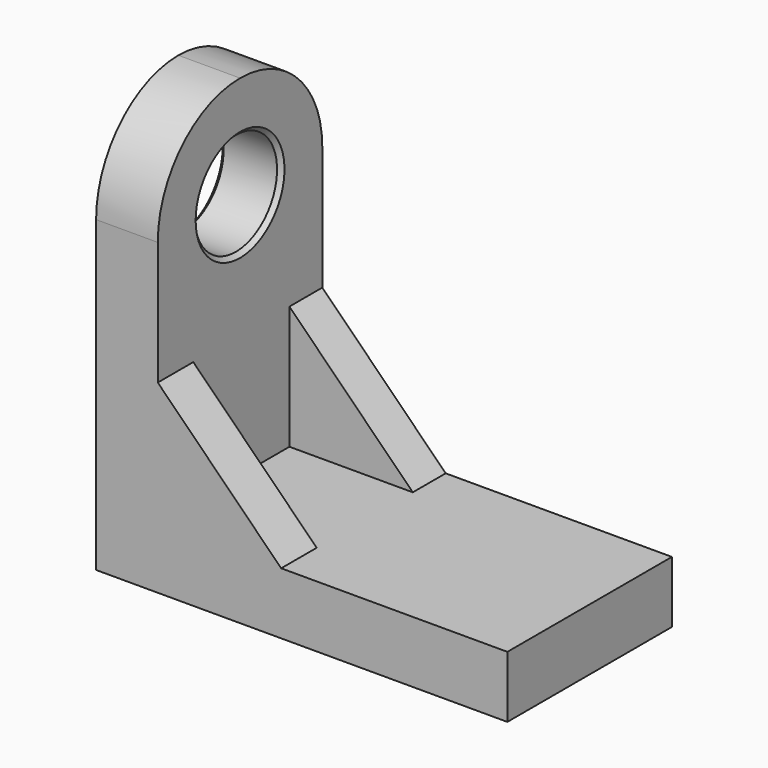
from build123d import *

# Parameters (mm, degrees)
F0_W     = 100
F0_H     = 50
F1_DEPTH = 15
F2_W     = 15
F2_H     = 50
F3_DEPTH = 85
F4_W     = 30
F4_H     = 10.7893505692
F4_H_2   = 10
F5_DEPTH = 30
F6_SIZE  = 29.99999
F7_R     = 12.5
F8_R     = 12.5
F9_DEPTH = 25
F10_R    = 24.99999
F11_SIZE = 1


# Not quite as in the source:
# - a fillet or chamfer is up to 0.001 mm smaller than in the source, because OpenCascade refuses the exact size


with BuildPart() as f1:
    # F0 (on Top) → F1 (new body)
    with BuildSketch(Plane.XY):
        with Locations((1.2109465897, -8.8487002536)):
            Rectangle(F0_W, F0_H)
    extrude(amount=F1_DEPTH)

    # F2 (on face) → F3 (join)
    with BuildSketch(Plane.XY.offset(15)):
        with Locations((-41.2890534103, -8.8487002536)):
            Rectangle(F2_W, F2_H)
    extrude(amount=F3_DEPTH)

    # F4 (on face) → F5 (join)
    with BuildSketch(Plane.XY.offset(15)):
        with Locations((-18.7890534103, -28.454024969)):
            Rectangle(F4_W, F4_H)
        with Locations((-18.7890534103, 11.1512997464)):
            Rectangle(F4_W, F4_H_2)
    extrude(amount=F5_DEPTH)

    # F6 (size 30 in the source; OpenCascade refuses exactly that, so slightly less here)
    f6_edges = [f1.edges().sort_by_distance(p)[0] for p in [
        (-3.789053, 11.1513, 45),
        (-3.789053, -28.454025, 45),
    ]]
    chamfer(f6_edges, length=F6_SIZE)

    # F7 (on face) + F8 (on face) → F9 (cut)
    with BuildSketch(Plane(origin=(-48.7890534103, 0, 0), x_dir=(0, -1, 0), z_dir=(-1, 0, 0))):
        with Locations((8.8487002536, 75)):
            Circle(F7_R)
    with BuildSketch(Plane(origin=(-48.7890534103, 0, 0), x_dir=(0, -1, 0), z_dir=(-1, 0, 0))):
        with Locations((8.8487002536, 75)):
            Circle(F8_R)
    extrude(amount=-F9_DEPTH, mode=Mode.SUBTRACT)

    # F10 (radius 25 in the source; OpenCascade refuses exactly that, so slightly less here)
    f10_edges = [f1.edges().sort_by_distance(p)[0] for p in [
        (-41.289053, 16.1513, 100),
        (-41.289053, -33.8487, 100),
    ]]
    fillet(f10_edges, radius=F10_R)

    # F11
    f11_edges = [f1.edges().sort_by_distance(p)[0] for p in [
        (-33.789053, 3.6513, 75),
        (-48.789053, 3.6513, 75),
    ]]
    chamfer(f11_edges, length=F11_SIZE)


solid = f1.part
